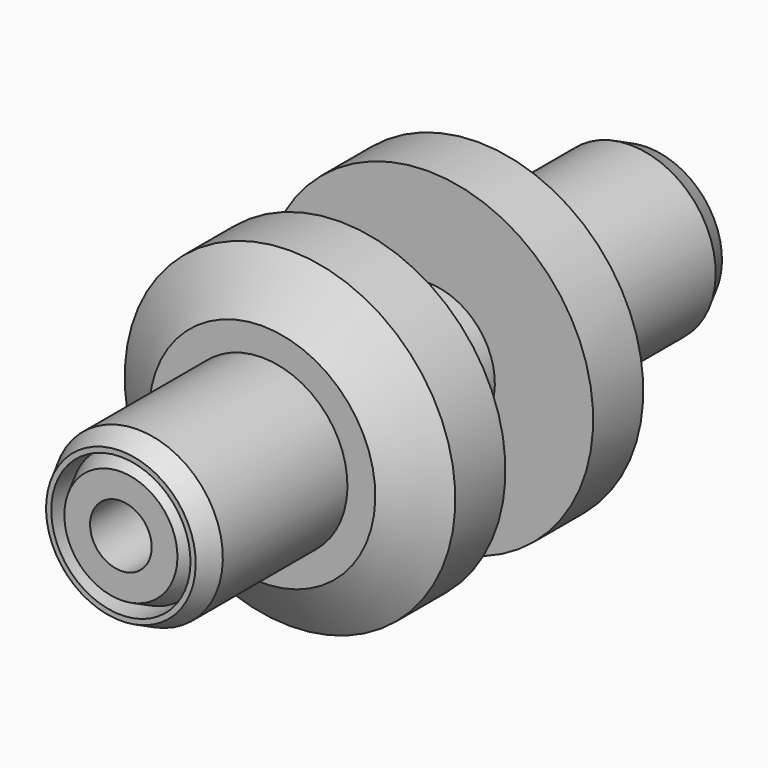
from build123d import *

# Parameters (mm, degrees)
F2_SIZE2   = 0.3
F2_SIZE    = 0.6
F2_2_SIZE2 = 0.3
F2_2_SIZE  = 0.6
F2_3_SIZE2 = 0.3
F2_3_SIZE  = 0.6


# Not quite as in the source:
# - a fillet or chamfer that OpenCascade refuses, or shapes differently, is made with other operations: its cross-section is extruded or revolved along the edge and cut away or added
# - two fillets or chamfers of one size are made in one step


with BuildPart() as f1:
    # F0 (on Right) → F1 (revolve)
    with BuildSketch(Plane.YZ):
        Polygon((-18.9, 1.925), (-18.9, 0.885), (0, 0.885), (0, 2.45), (-5.075, 2.45), (-5.075, 4.75), (-7.875, 4.75), (-7.875, 1.925), align=None)
    revolve(axis=Axis((0, -9.45, 0), (0, -1, 0)))

    # F2
    f2_edges = [f1.edges().sort_by_distance(p)[0] for p in [
        (0, -18.9, -1.925),
    ]]
    f2_side = f1.faces().sort_by_distance((0, -13.3875, -1.925))[0]
    chamfer(f2_edges, length=F2_SIZE, length2=F2_SIZE2, reference=f2_side)

    # F2#2
    f2_2_edges = [f1.edges().sort_by_distance(p)[0] for p in [
        (0, 0, -2.45),
    ]]
    f2_2_side = f1.faces().sort_by_distance((0, -2.5375, -2.45))[0]
    chamfer(f2_2_edges, length=F2_2_SIZE, length2=F2_2_SIZE2, reference=f2_2_side)

    # F4#2: chamfer of 1 x 1.5 on 1 edges, made by hand

    # F4_2_s1 → F4_2_t2 (revolve, cut)
    with BuildSketch(Plane.YZ):
        Polygon((-5.075, 3.25), (-6.075, 4.75), (-5.075, 4.75), align=None)
    revolve(axis=Axis((0, -5.075, 0), (0, -1, 0)), mode=Mode.SUBTRACT)


with BuildPart() as f1b:
    # F0 (on Right) → F1, piece 2 (revolve)
    with BuildSketch(Plane.YZ):
        Polygon((-18.9, 2.45), (-18.9, 2), (-11.025, 2), (-11.025, 4.75), (-13.825, 4.75), (-13.825, 2.45), align=None)
    revolve(axis=Axis((0, -9.45, 0), (0, -1, 0)))

    # F2#3
    f2_3_edges = [f1b.edges().sort_by_distance(p)[0] for p in [
        (0, -18.9, -2.45),
    ]]
    f2_3_side = f1b.faces().sort_by_distance((0, -16.3625, -2.45))[0]
    chamfer(f2_3_edges, length=F2_3_SIZE, length2=F2_3_SIZE2, reference=f2_3_side)

    # F4: chamfer of 1 x 1.5 on 1 edges, made by hand

    # F4_s1 → F4_t2 (revolve, cut)
    with BuildSketch(Plane.YZ):
        Polygon((-13.825, 3.25), (-12.825, 4.75), (-13.825, 4.75), align=None)
    revolve(axis=Axis((0, -13.825, 0), (0, -1, 0)), mode=Mode.SUBTRACT)


solid = Compound([f1.part, f1b.part])
